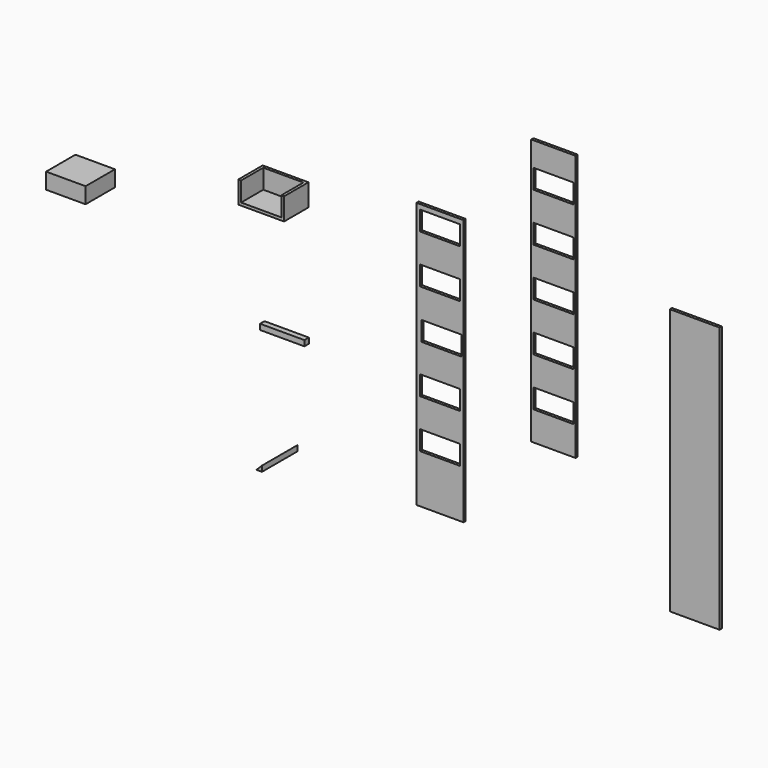
from build123d import *

# Parameters (mm, degrees)
F0_W      = 215.9
F0_H      = 1219.2
F0_W_2    = 184.15
F0_H_2    = 88.9
F1_DEPTH  = 12.7
F2_W      = 203.2
F2_H      = 1219.2
F2_W_2    = 184.15
F2_H_2    = 88.9
F3_DEPTH  = 12.7
F4_W      = 209.55
F4_H      = 101.6
F5_DEPTH  = 139.7
F6_W      = 184.15
F6_H      = 127
F7_DEPTH  = 88.9
F8_W      = 203.2
F8_H      = 25.4
F10_DEPTH = 25.4
F9_W      = 180.975
F9_H      = 73.025
F11_DEPTH = 168.275
F12_W     = 228.6
F12_H     = 1219.2
F13_DEPTH = 12.7
F15_DEPTH = 203.2


# Not quite as in the source:
# - a feature names something its author has since deleted; it is built from what else it names


with BuildPart() as f1:
    # F0 (on Front) → F1 (new body)
    with BuildSketch(Plane.XZ):
        with Locations((-107.95, 609.6)):
            Rectangle(F0_W, F0_H)
        with Locations((-107.95, 266.954)):
            Rectangle(F0_W_2, F0_H_2, mode=Mode.SUBTRACT)
        with Locations((-107.95, 488.442)):
            Rectangle(F0_W_2, F0_H_2, mode=Mode.SUBTRACT)
        with Locations((-101.6, 709.93)):
            Rectangle(F0_W_2, F0_H_2, mode=Mode.SUBTRACT)
        with Locations((-107.95, 931.418)):
            Rectangle(F0_W_2, F0_H_2, mode=Mode.SUBTRACT)
        with Locations((-107.95, 1152.906)):
            Rectangle(F0_W_2, F0_H_2, mode=Mode.SUBTRACT)
    extrude(amount=F1_DEPTH)


with BuildPart() as f3:
    # F2 (on Front) → F3 (new body)
    with BuildSketch(Plane.XZ):
        with Locations((411.6813279688, 1036.1642371192)):
            Rectangle(F2_W, F2_H)
        with Locations((411.6813279688, 604.6182371192)):
            Rectangle(F2_W_2, F2_H_2, mode=Mode.SUBTRACT)
        with Locations((411.6813279688, 826.1062371192)):
            Rectangle(F2_W_2, F2_H_2, mode=Mode.SUBTRACT)
        with Locations((411.6813279688, 1047.5942371192)):
            Rectangle(F2_W_2, F2_H_2, mode=Mode.SUBTRACT)
        with Locations((411.6813279688, 1269.0822371192)):
            Rectangle(F2_W_2, F2_H_2, mode=Mode.SUBTRACT)
        with Locations((411.6813279688, 1490.5702371192)):
            Rectangle(F2_W_2, F2_H_2, mode=Mode.SUBTRACT)
    extrude(amount=F3_DEPTH)


with BuildPart() as f5:
    # F4 (on Front) → F5 (new body)
    with BuildSketch(Plane.XZ):
        with Locations((-825.7857475758, 1081.6975569915)):
            Rectangle(F4_W, F4_H)
    extrude(amount=F5_DEPTH)

    # F6 (on face) → F7 (cut)
    with BuildSketch(Plane.XY.offset(1132.4975569915)):
        with Locations((-825.7857475758, -76.2)):
            Rectangle(F6_W, F6_H)
    extrude(amount=-F7_DEPTH, mode=Mode.SUBTRACT)


with BuildPart() as f10:
    # F8 (on Front) → F10 (new body)
    with BuildSketch(Plane.XZ):
        with Locations((-820.838779211, 493.9609521501)):
            Rectangle(F8_W, F8_H)
    extrude(amount=F10_DEPTH)


with BuildPart() as f11:
    # F9 (on Front) → F11 (new body)
    with BuildSketch(Plane.XZ):
        with Locations((-1698.2888811625, 860.1219307423)):
            Rectangle(F9_W, F9_H)
    extrude(amount=F11_DEPTH)


with BuildPart() as f13:
    # F12 (on Front) → F13 (new body)
    with BuildSketch(Plane.XZ):
        with Locations((1059.7636188984, 557.7803601671)):
            Rectangle(F12_W, F12_H)
    extrude(amount=F13_DEPTH)


with BuildPart() as f15:
    # F14 (on Front) → F15 (new body)
    with BuildSketch(Plane.XZ):
        Polygon((-771.3568039894, 30.289914459), (-771.3568039894, 55.689914459), (-796.7568039894, 30.289914459), align=None)
    extrude(amount=F15_DEPTH)


solid = Compound([f1.part, f3.part, f5.part, f10.part, f11.part, f13.part, f15.part])
